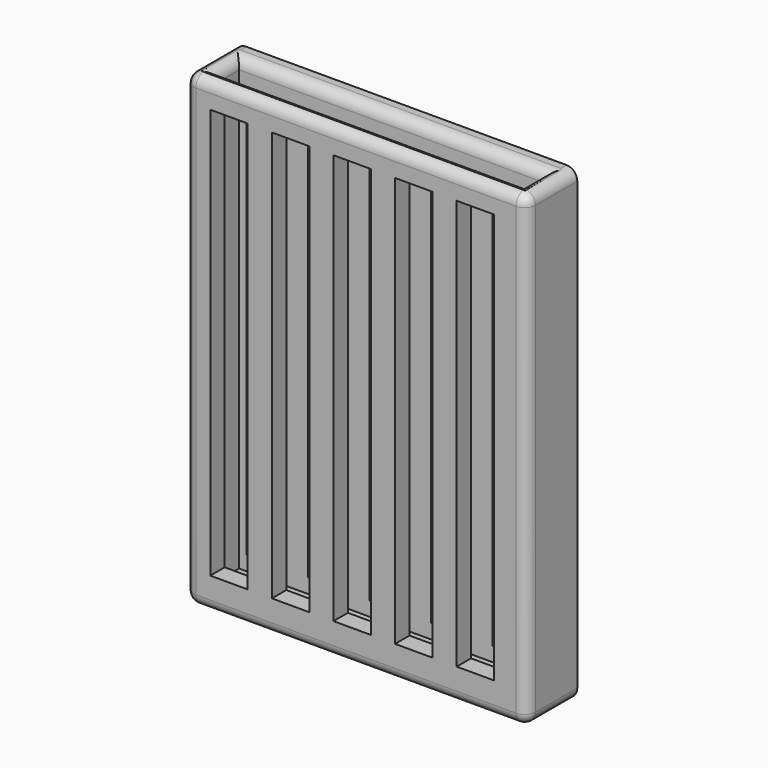
from build123d import *

# Parameters (mm, degrees)
F0_W         = 120.65
F0_H         = 22.225
F0_W_2       = 107.95
F0_H_2       = 9.525
F1_DEPTH     = 165.1
F2_W         = 22.225
F2_H         = 6.35
F3_DEPTH     = 55.88
F5_T1_DEPTH  = 113.03
F5_T3_DEPTH  = 27.94
F5_T5_DEPTH  = 157.48
F5_T7_DEPTH  = 9.525
F5_T9_DEPTH  = 107.95
F5_S13_W     = 3.81
F5_S13_H     = 3.81
F5_T14_DEPTH = 3.81
F5_S19_W     = 3.81
F5_S19_H     = 3.81
F5_T20_DEPTH = 3.81
F5_S25_W     = 3.81
F5_S25_H     = 3.81
F5_T26_DEPTH = 3.81
F5_S31_W     = 3.81
F5_S31_H     = 3.81
F5_T32_DEPTH = 3.81
F5_T39_DEPTH = 117.475
F5_T43_DEPTH = 19.05
F5_T50_DEPTH = 19.05
F5_T54_DEPTH = 117.475
F5_T61_DEPTH = 19.05
F5_T65_DEPTH = 117.475
F5_T72_DEPTH = 19.05
F5_T76_DEPTH = 117.475
F4_W         = 13.208
F4_H         = 144.78
F6_DEPTH     = 40.64


# Not quite as in the source:
# - a fillet or chamfer that OpenCascade refuses, or shapes differently, is made with other operations: its cross-section is extruded or revolved along the edge and cut away or added
# - a feature names something its author has since deleted; it is built from what else it names


with BuildPart() as f1:
    # F0 (on Top) → F1 (new body)
    with BuildSketch(Plane.XY):
        Rectangle(F0_W, F0_H)
        Rectangle(F0_W_2, F0_H_2, mode=Mode.SUBTRACT)
    extrude(amount=F1_DEPTH)

    # F2 (on Right) → F3 (join, symmetric)
    with BuildSketch(Plane.YZ):
        with Locations((0, 3.175)):
            Rectangle(F2_W, F2_H)
    extrude(amount=F3_DEPTH, both=True)

    # F5: fillet of radius 3.81 on 12 edges, made by hand

    # F5_s2 → F5_t1 (cut)
    with BuildSketch(Plane.YZ.offset(-56.515)):
        with BuildLine():
            ThreePointArc((-11.1125, 161.29), (-9.9965768363, 163.9840768363), (-7.3025, 165.1))
            Line((-7.3025, 165.1), (-11.1125, 165.1))
            Line((-11.1125, 165.1), (-11.1125, 161.29))
        make_face()
        with BuildLine():
            ThreePointArc((-11.1125, 3.81), (-9.9965768363, 1.1159231637), (-7.3025, 0))
            Line((-7.3025, 0), (-11.1125, 0))
            Line((-11.1125, 0), (-11.1125, 3.81))
        make_face()
    extrude(amount=F5_T1_DEPTH, mode=Mode.SUBTRACT)

    # F5_s4 → F5_t3 (cut)
    with BuildSketch(Plane.XZ.offset(-20.6375)):
        with BuildLine():
            ThreePointArc((-60.325, 161.29), (-59.2090768363, 163.9840768363), (-56.515, 165.1))
            Line((-56.515, 165.1), (-60.325, 165.1))
            Line((-60.325, 165.1), (-60.325, 161.29))
        make_face()
        with BuildLine():
            ThreePointArc((56.515, 165.1), (59.2090768363, 163.9840768363), (60.325, 161.29))
            Line((60.325, 161.29), (60.325, 165.1))
            Line((60.325, 165.1), (56.515, 165.1))
        make_face()
        with BuildLine():
            ThreePointArc((60.325, 3.81), (59.2090768363, 1.1159231637), (56.515, 0))
            Line((56.515, 0), (60.325, 0))
            Line((60.325, 0), (60.325, 3.81))
        make_face()
        with BuildLine():
            ThreePointArc((-60.325, 3.81), (-59.2090768363, 1.1159231637), (-56.515, 0))
            Line((-56.515, 0), (-60.325, 0))
            Line((-60.325, 0), (-60.325, 3.81))
        make_face()
    extrude(amount=F5_T3_DEPTH, mode=Mode.SUBTRACT)

    # F5_s6 → F5_t5 (cut)
    with BuildSketch(Plane.XY.offset(3.81)):
        with BuildLine():
            ThreePointArc((56.515, -11.1125), (59.2090768363, -9.9965768363), (60.325, -7.3025))
            Line((60.325, -7.3025), (60.325, -11.1125))
            Line((60.325, -11.1125), (56.515, -11.1125))
        make_face()
        with BuildLine():
            ThreePointArc((-60.325, -7.3025), (-59.2090768363, -9.9965768363), (-56.515, -11.1125))
            Line((-56.515, -11.1125), (-60.325, -11.1125))
            Line((-60.325, -11.1125), (-60.325, -7.3025))
        make_face()
    extrude(amount=F5_T5_DEPTH, mode=Mode.SUBTRACT)

    # F5_s8 → F5_t7 (cut)
    with BuildSketch(Plane.XZ.offset(-4.7625)):
        with BuildLine():
            ThreePointArc((57.785, 165.1), (55.0909231637, 163.9840768363), (53.975, 161.29))
            Line((53.975, 161.29), (53.975, 165.1))
            Line((53.975, 165.1), (57.785, 165.1))
        make_face()
        with BuildLine():
            ThreePointArc((-57.785, 165.1), (-55.0909231637, 163.9840768363), (-53.975, 161.29))
            Line((-53.975, 161.29), (-53.975, 165.1))
            Line((-53.975, 165.1), (-57.785, 165.1))
        make_face()
    extrude(amount=F5_T7_DEPTH, mode=Mode.SUBTRACT)

    # F5_s10 → F5_t9 (cut)
    with BuildSketch(Plane.YZ.offset(-53.975)):
        with BuildLine():
            ThreePointArc((-8.5725, 165.1), (-5.8784231637, 163.9840768363), (-4.7625, 161.29))
            Line((-4.7625, 161.29), (-4.7625, 165.1))
            Line((-4.7625, 165.1), (-8.5725, 165.1))
        make_face()
        with BuildLine():
            ThreePointArc((8.5725, 165.1), (5.8784231637, 163.9840768363), (4.7625, 161.29))
            Line((4.7625, 161.29), (4.7625, 165.1))
            Line((4.7625, 165.1), (8.5725, 165.1))
        make_face()
    extrude(amount=F5_T9_DEPTH, mode=Mode.SUBTRACT)


with BuildPart() as f5_tool12:
    # F5_s13 → F5_t14 (new body)
    with BuildSketch(Plane.YZ.offset(-56.515)):
        with Locations((-9.2075, 163.195)):
            Rectangle(F5_S13_W, F5_S13_H)
    extrude(amount=-F5_T14_DEPTH)

    # F5_s15 → F5_t16 (revolve, cut)
    with BuildSketch(Plane(origin=(-56.515, -7.3025, 161.29), x_dir=(0, 0.7071067812, -0.7071067812), z_dir=(0, 0.7071067812, 0.7071067812))):
        with BuildLine():
            ThreePointArc((0, -3.81), (3.81, 0), (0, 3.81))
            Line((0, 3.81), (0, -3.81))
        make_face()
    revolve(axis=Axis((-56.515, -7.3025, 161.29), (-1, 0, 0)), mode=Mode.SUBTRACT)


with BuildPart() as f1_1:
    add(f1.part)

    # F5_t11: cut F5_tool12
    add(f5_tool12.part, mode=Mode.SUBTRACT)


with BuildPart() as f5_tool18:
    # F5_s19 → F5_t20 (new body)
    with BuildSketch(Plane.YZ.offset(56.515)):
        with Locations((-9.2075, 163.195)):
            Rectangle(F5_S19_W, F5_S19_H)
    extrude(amount=F5_T20_DEPTH)

    # F5_s21 → F5_t22 (revolve, cut)
    with BuildSketch(Plane(origin=(56.515, -7.3025, 161.29), x_dir=(0, 0.7071067812, -0.7071067812), z_dir=(0, -0.7071067812, -0.7071067812))):
        with BuildLine():
            ThreePointArc((0, -3.81), (3.81, 0), (0, 3.81))
            Line((0, 3.81), (0, -3.81))
        make_face()
    revolve(axis=Axis((56.515, -7.3025, 161.29), (1, 0, 0)), mode=Mode.SUBTRACT)


with BuildPart() as f1_2:
    add(f1_1.part)

    # F5_t17: cut F5_tool18
    add(f5_tool18.part, mode=Mode.SUBTRACT)


with BuildPart() as f5_tool24:
    # F5_s25 → F5_t26 (new body)
    with BuildSketch(Plane.YZ.offset(56.515)):
        with Locations((-9.2075, 1.905)):
            Rectangle(F5_S25_W, F5_S25_H)
    extrude(amount=F5_T26_DEPTH)

    # F5_s27 → F5_t28 (revolve, cut)
    with BuildSketch(Plane(origin=(56.515, -7.3025, 3.81), x_dir=(0, 0.7071067812, 0.7071067812), z_dir=(0, 0.7071067812, -0.7071067812))):
        with BuildLine():
            ThreePointArc((0, -3.81), (3.81, 0), (0, 3.81))
            Line((0, 3.81), (0, -3.81))
        make_face()
    revolve(axis=Axis((56.515, -7.3025, 3.81), (1, 0, 0)), mode=Mode.SUBTRACT)


with BuildPart() as f1_3:
    add(f1_2.part)

    # F5_t23: cut F5_tool24
    add(f5_tool24.part, mode=Mode.SUBTRACT)


with BuildPart() as f5_tool30:
    # F5_s31 → F5_t32 (new body)
    with BuildSketch(Plane.YZ.offset(-56.515)):
        with Locations((-9.2075, 1.905)):
            Rectangle(F5_S31_W, F5_S31_H)
    extrude(amount=-F5_T32_DEPTH)

    # F5_s33 → F5_t34 (revolve, cut)
    with BuildSketch(Plane(origin=(-56.515, -7.3025, 3.81), x_dir=(0, 0.7071067812, 0.7071067812), z_dir=(0, -0.7071067812, 0.7071067812))):
        with BuildLine():
            ThreePointArc((0, -3.81), (3.81, 0), (0, 3.81))
            Line((0, 3.81), (0, -3.81))
        make_face()
    revolve(axis=Axis((-56.515, -7.3025, 3.81), (-1, 0, 0)), mode=Mode.SUBTRACT)


with BuildPart() as f1_4:
    add(f1_3.part)

    # F5_t29: cut F5_tool30
    add(f5_tool30.part, mode=Mode.SUBTRACT)


with BuildPart() as f5_tool37:
    # F5_s38 → F5_t39 (new body)
    with BuildSketch(Plane.YZ.offset(-53.975)):
        with BuildLine():
            ThreePointArc((8.5725, 165.1), (5.8784231637, 163.9840768363), (4.7625, 161.29))
            Line((4.7625, 161.29), (4.7625, 165.1))
            Line((4.7625, 165.1), (8.5725, 165.1))
        make_face()
    extrude(amount=F5_T39_DEPTH)

    split(bisect_by=Plane.YZ.offset(53.975), keep=Keep.TOP)


with BuildPart() as f5_tool41:
    # F5_s42 → F5_t43 (new body)
    with BuildSketch(Plane.XZ.offset(-14.2875)):
        with BuildLine():
            ThreePointArc((57.785, 165.1), (55.0909231637, 163.9840768363), (53.975, 161.29))
            Line((53.975, 161.29), (53.975, 165.1))
            Line((53.975, 165.1), (57.785, 165.1))
        make_face()
    extrude(amount=F5_T43_DEPTH)

    split(bisect_by=Plane.XZ.offset(-4.7625), keep=Keep.BOTTOM)


with BuildPart() as f5_tool37_1:
    add(f5_tool37.part)

    # F5_t45: intersect F5_tool41
    add(f5_tool41.part, mode=Mode.INTERSECT)


with BuildPart() as f1_5:
    add(f1_4.part)

    # F5_t35: cut F5_tool37
    add(f5_tool37_1.part, mode=Mode.SUBTRACT)


with BuildPart() as f5_tool48:
    # F5_s49 → F5_t50 (new body)
    with BuildSketch(Plane.XZ.offset(-4.7625)):
        with BuildLine():
            ThreePointArc((57.785, 165.1), (55.0909231637, 163.9840768363), (53.975, 161.29))
            Line((53.975, 161.29), (53.975, 165.1))
            Line((53.975, 165.1), (57.785, 165.1))
        make_face()
    extrude(amount=F5_T50_DEPTH)

    split(bisect_by=Plane.XZ.offset(4.7625), keep=Keep.TOP)


with BuildPart() as f5_tool52:
    # F5_s53 → F5_t54 (new body)
    with BuildSketch(Plane.YZ.offset(63.5)):
        with BuildLine():
            ThreePointArc((-8.5725, 165.1), (-5.8784231637, 163.9840768363), (-4.7625, 161.29))
            Line((-4.7625, 161.29), (-4.7625, 165.1))
            Line((-4.7625, 165.1), (-8.5725, 165.1))
        make_face()
    extrude(amount=-F5_T54_DEPTH)

    split(bisect_by=Plane.YZ.offset(53.975), keep=Keep.TOP)


with BuildPart() as f5_tool48_1:
    add(f5_tool48.part)

    # F5_t56: intersect F5_tool52
    add(f5_tool52.part, mode=Mode.INTERSECT)


with BuildPart() as f1_6:
    add(f1_5.part)

    # F5_t46: cut F5_tool48
    add(f5_tool48_1.part, mode=Mode.SUBTRACT)


with BuildPart() as f5_tool59:
    # F5_s60 → F5_t61 (new body)
    with BuildSketch(Plane.XZ.offset(14.2875)):
        with BuildLine():
            ThreePointArc((-57.785, 165.1), (-55.0909231637, 163.9840768363), (-53.975, 161.29))
            Line((-53.975, 161.29), (-53.975, 165.1))
            Line((-53.975, 165.1), (-57.785, 165.1))
        make_face()
    extrude(amount=-F5_T61_DEPTH)

    split(bisect_by=Plane.XZ.offset(4.7625), keep=Keep.TOP)


with BuildPart() as f5_tool63:
    # F5_s64 → F5_t65 (new body)
    with BuildSketch(Plane.YZ.offset(53.975)):
        with BuildLine():
            ThreePointArc((-8.5725, 165.1), (-5.8784231637, 163.9840768363), (-4.7625, 161.29))
            Line((-4.7625, 161.29), (-4.7625, 165.1))
            Line((-4.7625, 165.1), (-8.5725, 165.1))
        make_face()
    extrude(amount=-F5_T65_DEPTH)

    split(bisect_by=Plane.YZ.offset(-53.975), keep=Keep.BOTTOM)


with BuildPart() as f5_tool59_1:
    add(f5_tool59.part)

    # F5_t67: intersect F5_tool63
    add(f5_tool63.part, mode=Mode.INTERSECT)


with BuildPart() as f1_7:
    add(f1_6.part)

    # F5_t57: cut F5_tool59
    add(f5_tool59_1.part, mode=Mode.SUBTRACT)


with BuildPart() as f5_tool70:
    # F5_s71 → F5_t72 (new body)
    with BuildSketch(Plane.XZ.offset(4.7625)):
        with BuildLine():
            ThreePointArc((-57.785, 165.1), (-55.0909231637, 163.9840768363), (-53.975, 161.29))
            Line((-53.975, 161.29), (-53.975, 165.1))
            Line((-53.975, 165.1), (-57.785, 165.1))
        make_face()
    extrude(amount=-F5_T72_DEPTH)

    split(bisect_by=Plane.XZ.offset(-4.7625), keep=Keep.BOTTOM)


with BuildPart() as f5_tool74:
    # F5_s75 → F5_t76 (new body)
    with BuildSketch(Plane.YZ.offset(-63.5)):
        with BuildLine():
            ThreePointArc((8.5725, 165.1), (5.8784231637, 163.9840768363), (4.7625, 161.29))
            Line((4.7625, 161.29), (4.7625, 165.1))
            Line((4.7625, 165.1), (8.5725, 165.1))
        make_face()
    extrude(amount=F5_T76_DEPTH)

    split(bisect_by=Plane.YZ.offset(-53.975), keep=Keep.BOTTOM)


with BuildPart() as f5_tool70_1:
    add(f5_tool70.part)

    # F5_t78: intersect F5_tool74
    add(f5_tool74.part, mode=Mode.INTERSECT)


with BuildPart() as f1_8:
    add(f1_7.part)

    # F5_t68: cut F5_tool70
    add(f5_tool70_1.part, mode=Mode.SUBTRACT)

    # F4 (on face) → F6 (cut)
    with BuildSketch(Plane.XZ.offset(11.1125)):
        with Locations((-44.831, 83.82)):
            Rectangle(F4_W, F4_H)
        with Locations((-23.0886, 83.82)):
            Rectangle(F4_W, F4_H)
        with Locations((-1.3462, 83.82)):
            Rectangle(F4_W, F4_H)
        with Locations((20.3962, 83.82)):
            Rectangle(F4_W, F4_H)
        with Locations((42.1386, 83.82)):
            Rectangle(F4_W, F4_H)
    extrude(amount=-F6_DEPTH, mode=Mode.SUBTRACT)


solid = f1_8.part
